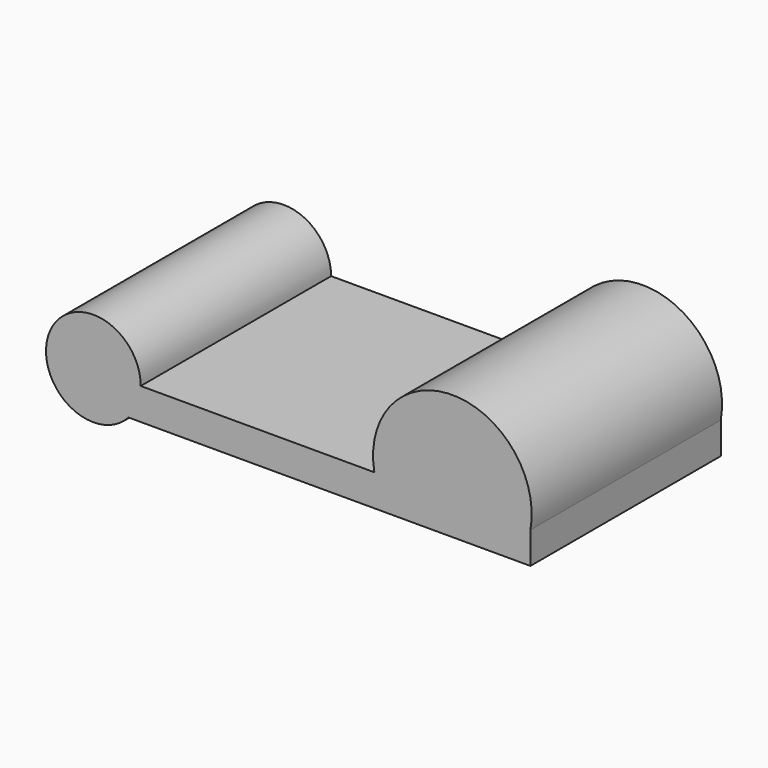
from build123d import *

# Parameters (mm, degrees)
F1_DEPTH = 38.1


# Not quite as in the source:
# - the program builds the solid bodies; features that only make, move or delete a surface that nothing else refers to are left out


with BuildPart() as f1:
    # F0 (on Front) → F1 (new body)
    with BuildSketch(Plane.XZ):
        with BuildLine():
            Line((-12.4957701793, -2.2684196318), (12.4957701793, -2.2684196318))
            ThreePointArc((12.4957701793, -2.2684196318), (0, 12.7), (-12.4957701793, -2.2684196318))
        make_face()
        with BuildLine():
            Line((12.4957701793, -7.3484196318), (12.4957701793, -2.2684196318))
            Line((12.4957701793, -2.2684196318), (-12.4957701793, -2.2684196318))
            Line((-12.4957701793, -2.2684196318), (-49.8945600124, -2.2684196318))
            ThreePointArc((-49.8945600124, -2.2684196318), (-50.3994056233, -4.9895144213), (-51.8467453044, -7.3484196318))
            Line((-51.8467453044, -7.3484196318), (12.4957701793, -7.3484196318))
        make_face()
        with BuildLine():
            ThreePointArc((-51.8467453044, -7.3484196318), (-50.3994056233, -4.9895144213), (-49.8945600124, -2.2684196318))
            Line((-49.8945600124, -2.2684196318), (-57.4802711475, -2.2684196318))
            Line((-57.4802711475, -2.2684196318), (-57.4802711475, -7.3484196318))
            Line((-57.4802711475, -7.3484196318), (-51.8467453044, -7.3484196318))
        make_face()
        with BuildLine():
            Line((-57.4802711475, -2.2684196318), (-49.8945600124, -2.2684196318))
            ThreePointArc((-49.8945600124, -2.2684196318), (-64.5611366718, 0.4526751578), (-51.8467453044, -7.3484196318))
            Line((-51.8467453044, -7.3484196318), (-57.4802711475, -7.3484196318))
            Line((-57.4802711475, -7.3484196318), (-57.4802711475, -2.2684196318))
        make_face()
    extrude(amount=F1_DEPTH)


solid = f1.part
